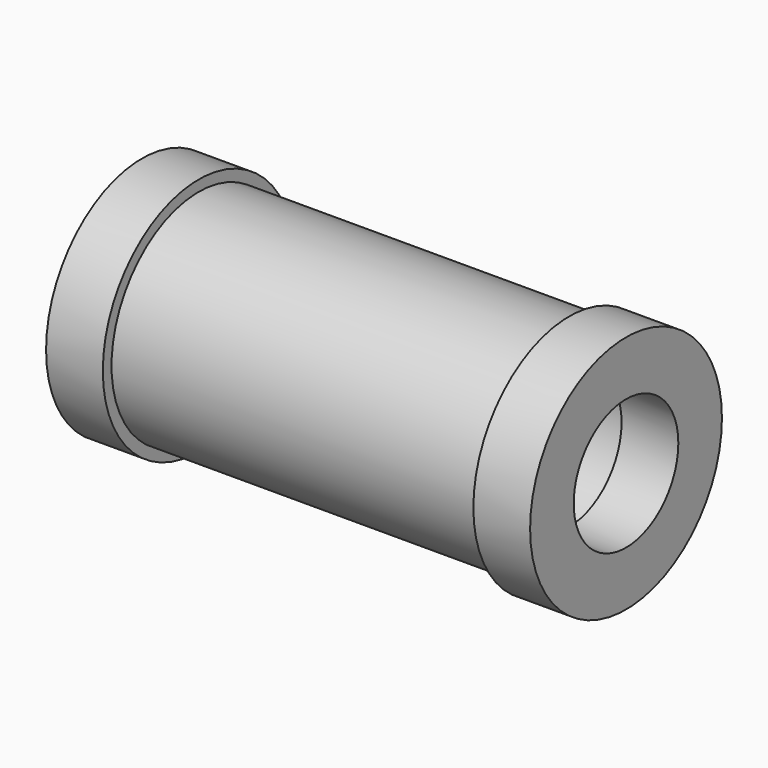
from build123d import *

# Parameters (mm, degrees)
F0_R     = 20
F0_R_2   = 15
F1_DEPTH = 34
F2_R     = 22
F2_R_2   = 12
F3_DEPTH = 10.414


# Not quite as in the source:
# - a pattern or mirror of a feature is missing from the dataset's text; its kind, count and spacing are read off the source's solid


with BuildPart() as f1:
    # F0 (on Right) → F1 (new body, symmetric)
    with BuildSketch(Plane.YZ):
        Circle(F0_R)
        Circle(F0_R_2, mode=Mode.SUBTRACT)
    extrude(amount=F1_DEPTH, both=True)

    # F2 (on face) → F3 (join)
    with BuildSketch(Plane.YZ.offset(34)):
        Circle(F2_R)
        Circle(F2_R_2, mode=Mode.SUBTRACT)
    f3 = extrude(amount=F3_DEPTH)

    # F3_copies: F3 across plane
    add(f3.mirror(Plane(origin=(0, 0, 0), x_dir=(0, 0, -1), z_dir=(-1, 0, 0))))


solid = f1.part
